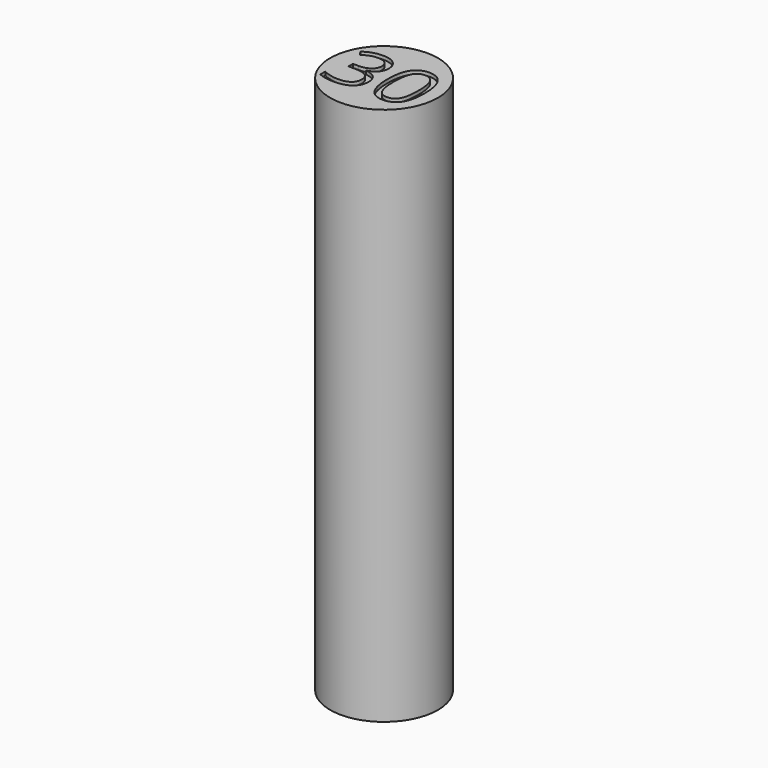
from build123d import *

# Parameters (mm, degrees)
F0_R         = 15
F1_DEPTH     = 150
F2_TEXT_SIZE = 22.2222222222
F3_DEPTH     = 1
F4_TEXT_SIZE = 22.2222222222
F5_DEPTH     = 1


# Not quite as in the source:
# - Text() gives the source's letters only with a copy of the font that has no kerning and outlines rounded to 1/6400 em; it was checked with that copy


with BuildPart() as f1:
    # F0 (on Top) → F1 (new body)
    with BuildSketch(Plane.XY):
        Circle(F0_R)
    extrude(amount=F1_DEPTH)

    # F2 (on face) → F3 (cut)
    with BuildSketch(Plane(origin=(0, 0, 0), x_dir=(1, 0, 0), z_dir=(0, 0, -1))):
        with Locations((-12.8732638889, -8)):
            Text('30', F2_TEXT_SIZE, font='Open Sans', text_align=(TextAlign.LEFT, TextAlign.BOTTOM))
    extrude(amount=-F3_DEPTH, mode=Mode.SUBTRACT)

    # F4 (on face) → F5 (cut)
    with BuildSketch(Plane.XY.offset(150)):
        with Locations((-12.8732638889, -8)):
            Text('30', F4_TEXT_SIZE, font='Open Sans', text_align=(TextAlign.LEFT, TextAlign.BOTTOM))
    extrude(amount=-F5_DEPTH, mode=Mode.SUBTRACT)


solid = f1.part
